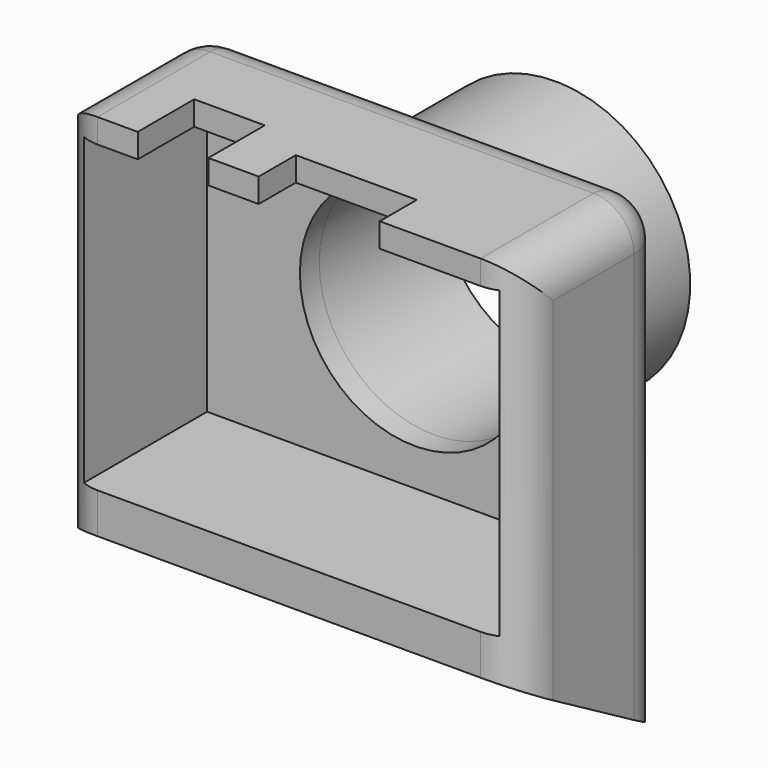
from build123d import *

# Parameters (mm, degrees)
F0_W          = 23
F0_H          = 17.5
F1_DEPTH      = 9
F2_T          = -1.2
F3_R          = 5.7
F4_DEPTH      = 3
F3_R_2        = 6.7
F5_DEPTH      = 7.5
F6_W          = 6
F6_H          = 2.3
F6_W_2        = 3.5
F6_H_2        = 3.5
F7_DEPTH      = 4
F8_DEPTH      = 6
F10_DEPTH     = 30
F11_T1_DEPTH  = 19
F11_T3_DEPTH  = 26.5
F11_T5_DEPTH  = 12
F11_T7_DEPTH  = 28.3038475773
F11_S11_W     = 2
F11_S11_H     = 2
F11_T12_DEPTH = 2
F11_S17_W     = 2
F11_S17_H     = 2
F11_T18_DEPTH = 2


# Not quite as in the source:
# - a fillet or chamfer that OpenCascade refuses, or shapes differently, is made with other operations: its cross-section is extruded or revolved along the edge and cut away or added


with BuildPart() as f1:
    # F0 (on Front) → F1 (new body)
    with BuildSketch(Plane.XZ):
        Rectangle(F0_W, F0_H)
    extrude(amount=F1_DEPTH)

    # F2
    f2_openings = [f1.faces().sort_by_distance(p)[0] for p in [
        (0, -9, 0),
    ]]
    offset(amount=F2_T, openings=f2_openings)

    # F3 (on face) → F4 (cut)
    with BuildSketch(Plane(origin=(0, 0, 0), x_dir=(-1, 0, 0), z_dir=(0, 1, 0))):
        Circle(F3_R)
    extrude(amount=-F4_DEPTH, mode=Mode.SUBTRACT)

    # F3 (on face) → F5 (join)
    with BuildSketch(Plane(origin=(0, 0, 0), x_dir=(-1, 0, 0), z_dir=(0, 1, 0))):
        Circle(F3_R_2)
        Circle(F3_R, mode=Mode.SUBTRACT)
    extrude(amount=F5_DEPTH)

    # F6 (on face) → F7 (cut)
    with BuildSketch(Plane.XY.offset(8.75)):
        with Locations((1.5, -7.85)):
            Rectangle(F6_W, F6_H)
        with Locations((-5.75, -7.25)):
            Rectangle(F6_W_2, F6_H_2)
    extrude(amount=-F7_DEPTH, mode=Mode.SUBTRACT)

    # F8 (add): a face of the model
    f8_faces = [f1.faces().sort_by_distance(p)[0] for p in [
        (0, -4.5, -8.75),
    ]]
    extrude(f8_faces, amount=F8_DEPTH)

    # F9 (on face) → F10 (cut)
    with BuildSketch(Plane.YZ.offset(11.5)):
        Polygon((-9, -14.75), (0, -14.75), (-9, -9.5538475773), align=None)
    extrude(amount=-F10_DEPTH, mode=Mode.SUBTRACT)

    # F11: fillet of radius 2 on 7 edges, made by hand

    # F11_s2 → F11_t1 (cut)
    with BuildSketch(Plane.YZ.offset(-9.5)):
        with BuildLine():
            ThreePointArc((0, 6.75), (-0.5857864376, 8.1642135624), (-2, 8.75))
            Line((-2, 8.75), (0, 8.75))
            Line((0, 8.75), (0, 6.75))
        make_face()
    extrude(amount=F11_T1_DEPTH, mode=Mode.SUBTRACT)

    # F11_s4 → F11_t3 (cut)
    with BuildSketch(Plane.XY.offset(-19.75)):
        with BuildLine():
            ThreePointArc((-11.5, -2), (-10.9142135624, -0.5857864376), (-9.5, 0))
            Line((-9.5, 0), (-11.5, 0))
            Line((-11.5, 0), (-11.5, -2))
        make_face()
        with BuildLine():
            ThreePointArc((9.5, 0), (10.9142135624, -0.5857864376), (11.5, -2))
            Line((11.5, -2), (11.5, 0))
            Line((11.5, 0), (9.5, 0))
        make_face()
    extrude(amount=F11_T3_DEPTH, mode=Mode.SUBTRACT)

    # F11_s6 → F11_t5 (cut)
    with BuildSketch(Plane.XZ.offset(2)):
        with BuildLine():
            ThreePointArc((9.5, 8.75), (10.9142135624, 8.1642135624), (11.5, 6.75))
            Line((11.5, 6.75), (11.5, 8.75))
            Line((11.5, 8.75), (9.5, 8.75))
        make_face()
        with BuildLine():
            ThreePointArc((-11.5, 6.75), (-10.9142135624, 8.1642135624), (-9.5, 8.75))
            Line((-9.5, 8.75), (-11.5, 8.75))
            Line((-11.5, 8.75), (-11.5, 6.75))
        make_face()
    extrude(amount=F11_T5_DEPTH, mode=Mode.SUBTRACT)

    # F11_s8 → F11_t7 (cut)
    with BuildSketch(Plane.XY.offset(-14.5538475773)):
        with BuildLine():
            ThreePointArc((-11.5, -7), (-10.9142135624, -8.4142135624), (-9.5, -9))
            Line((-9.5, -9), (-11.5, -9))
            Line((-11.5, -9), (-11.5, -7))
        make_face()
        with BuildLine():
            ThreePointArc((9.5, -9), (10.9142135624, -8.4142135624), (11.5, -7))
            Line((11.5, -7), (11.5, -9))
            Line((11.5, -9), (9.5, -9))
        make_face()
    extrude(amount=F11_T7_DEPTH, mode=Mode.SUBTRACT)


with BuildPart() as f11_tool10:
    # F11_s11 → F11_t12 (new body)
    with BuildSketch(Plane.XZ.offset(2)):
        with Locations((10.5, 7.75)):
            Rectangle(F11_S11_W, F11_S11_H)
    extrude(amount=-F11_T12_DEPTH)

    # F11_s13 → F11_t14 (revolve, cut)
    with BuildSketch(Plane(origin=(9.5, -2, 6.75), x_dir=(-0.7071067812, 0, -0.7071067812), z_dir=(0.7071067812, 0, -0.7071067812))):
        with BuildLine():
            ThreePointArc((0, -2), (2, 0), (0, 2))
            Line((0, 2), (0, -2))
        make_face()
    revolve(axis=Axis((9.5, -2, 6.75), (0, 1, 0)), mode=Mode.SUBTRACT)


with BuildPart() as f1_1:
    add(f1.part)

    # F11_t9: cut F11_tool10
    add(f11_tool10.part, mode=Mode.SUBTRACT)


with BuildPart() as f11_tool16:
    # F11_s17 → F11_t18 (new body)
    with BuildSketch(Plane.YZ.offset(-9.5)):
        with Locations((-1, 7.75)):
            Rectangle(F11_S17_W, F11_S17_H)
    extrude(amount=-F11_T18_DEPTH)

    # F11_s19 → F11_t20 (revolve, cut)
    with BuildSketch(Plane(origin=(-9.5, -2, 6.75), x_dir=(0, -0.7071067812, -0.7071067812), z_dir=(0, 0.7071067812, -0.7071067812))):
        with BuildLine():
            ThreePointArc((0, -2), (2, 0), (0, 2))
            Line((0, 2), (0, -2))
        make_face()
    revolve(axis=Axis((-9.5, -2, 6.75), (-1, 0, 0)), mode=Mode.SUBTRACT)


with BuildPart() as f1_2:
    add(f1_1.part)

    # F11_t15: cut F11_tool16
    add(f11_tool16.part, mode=Mode.SUBTRACT)


solid = f1_2.part
